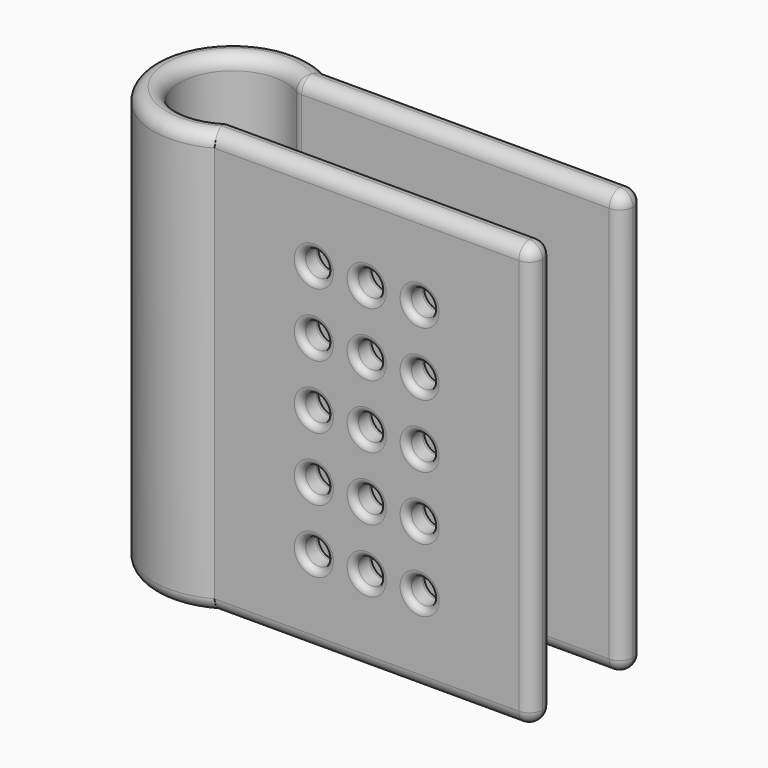
from build123d import *

# Parameters (mm, degrees)
F1_DEPTH = 25.4
F2_R     = 0.79374
F3_R     = 0.79375
F4_DEPTH = 8.9518078406
F5_R     = 0.381


# Not quite as in the source:
# - a fillet or chamfer is up to 0.001 mm smaller than in the source, because OpenCascade refuses the exact size


with BuildPart() as f1:
    # F0 (on Top) → F1 (new body)
    with BuildSketch(Plane.XY):
        with BuildLine():
            ThreePointArc((1.8211051854, -2.6008077406), (-3.175, 0), (1.8211051854, 2.6008077406))
            Line((1.8211051854, 2.6008077406), (2.7316577781, 3.9012116109))
            ThreePointArc((2.7316577781, 3.9012116109), (2.5034693369, 4.0514253701), (2.2670431226, 4.1883077406))
            ThreePointArc((2.2670431226, 4.1883077406), (-4.7625, 0), (2.2670431226, -4.1883077406))
            ThreePointArc((2.2670431226, -4.1883077406), (2.5034693369, -4.0514253701), (2.7316577781, -3.9012116109))
            Line((2.7316577781, -3.9012116109), (1.8211051854, -2.6008077406))
        make_face()
        with BuildLine():
            ThreePointArc((2.2670431226, 4.1883077406), (2.5034693369, 4.0514253701), (2.7316577781, 3.9012116109))
            ThreePointArc((2.7316577781, 3.9012116109), (3.4229686317, 3.3112976303), (3.989637245, 2.6008077406))
            Line((3.989637245, 2.6008077406), (21.3170431226, 2.6008077406))
            Line((21.3170431226, 2.6008077406), (21.3170431226, 4.1883077406))
            Line((21.3170431226, 4.1883077406), (2.2670431226, 4.1883077406))
        make_face()
        with BuildLine():
            Line((3.989637245, -2.6008077406), (1.8211051854, -2.6008077406))
            Line((1.8211051854, -2.6008077406), (2.7316577781, -3.9012116109))
            ThreePointArc((2.7316577781, -3.9012116109), (3.4229686317, -3.3112976303), (3.989637245, -2.6008077406))
        make_face()
        with BuildLine():
            ThreePointArc((3.989637245, -2.6008077406), (3.4229686317, -3.3112976303), (2.7316577781, -3.9012116109))
            ThreePointArc((2.7316577781, -3.9012116109), (2.5034693369, -4.0514253701), (2.2670431226, -4.1883077406))
            Line((2.2670431226, -4.1883077406), (21.3170431226, -4.1883077406))
            Line((21.3170431226, -4.1883077406), (21.3170431226, -2.6008077406))
            Line((21.3170431226, -2.6008077406), (3.989637245, -2.6008077406))
        make_face()
        with BuildLine():
            Line((2.7316577781, 3.9012116109), (1.8211051854, 2.6008077406))
            Line((1.8211051854, 2.6008077406), (3.989637245, 2.6008077406))
            ThreePointArc((3.989637245, 2.6008077406), (3.4229686317, 3.3112976303), (2.7316577781, 3.9012116109))
        make_face()
    extrude(amount=F1_DEPTH)

    # F2 (radius 0.79375 in the source; OpenCascade refuses exactly that, so slightly less here)
    f2_edges = [f1.edges().sort_by_distance(p)[0] for p in [
        (-3.175, 0, 25.4),
        (11.569074, 2.600808, 25.4),
        (21.317043, 3.394558, 25.4),
        (11.792043, 4.188308, 25.4),
        (-4.7625, 0, 25.4),
        (11.792043, -4.188308, 25.4),
        (21.317043, -3.394558, 25.4),
        (11.569074, -2.600808, 25.4),
        (-3.175, 0, 0),
        (11.569074, 2.600808, 0),
        (21.317043, 3.394558, 0),
        (11.792043, 4.188308, 0),
        (-4.7625, 0, 0),
        (11.792043, -4.188308, 0),
        (21.317043, -3.394558, 0),
        (11.569074, -2.600808, 0),
        (21.317043, 2.600808, 12.7),
        (21.317043, 4.188308, 12.7),
        (21.317043, -4.188308, 12.7),
        (21.317043, -2.600808, 12.7),
        (1.821105, -2.600808, 12.7),
        (1.821105, 2.600808, 12.7),
    ]]
    fillet(f2_edges, radius=F2_R)

    # F3 (on face) → F4 (cut, through all)
    with BuildSketch(Plane.XZ.offset(4.1883077406)):
        with Locations((11.3951681226, 12.7)):
            Circle(F3_R)
        with Locations((14.5701681226, 12.7000016774)):
            Circle(F3_R)
        with Locations((8.2201681226, 8.8900020029)):
            Circle(F3_R)
        with Locations((11.3951681226, 8.89)):
            Circle(F3_R)
        with Locations((14.5701681226, 8.8900016774)):
            Circle(F3_R)
        with Locations((11.3951681226, 5.08)):
            Circle(F3_R)
        with Locations((14.5701681226, 5.0800016774)):
            Circle(F3_R)
        with Locations((8.2201681226, 12.7000016774)):
            Circle(F3_R)
        with Locations((11.3951681226, 16.5100008387)):
            Circle(F3_R)
        with Locations((14.5701681226, 16.5100016774)):
            Circle(F3_R)
        with Locations((8.2201681226, 20.3200016774)):
            Circle(F3_R)
        with Locations((11.3951681226, 20.3200016774)):
            Circle(F3_R)
        with Locations((14.5701681226, 20.3200016774)):
            Circle(F3_R)
        with Locations((8.2201681226, 16.5100016774)):
            Circle(F3_R)
        with Locations((8.2201681226, 5.0800023283)):
            Circle(F3_R)
    extrude(amount=-F4_DEPTH, mode=Mode.SUBTRACT)

    # F5
    f5_edges = [f1.edges().sort_by_distance(p)[0] for p in [
        (7.426418, -4.188308, 5.080002),
        (9.013918, -3.394558, 5.080002),
        (7.426418, -2.600808, 5.080002),
        (7.426418, 2.600808, 5.080002),
        (9.013918, 3.394558, 5.080002),
        (7.426418, 4.188308, 5.080002),
        (10.601418, -4.188308, 5.08),
        (12.188918, -3.394558, 5.08),
        (10.601418, -2.600808, 5.08),
        (10.601418, 2.600808, 5.08),
        (12.188918, 3.394558, 5.08),
        (10.601418, 4.188308, 5.08),
        (13.776418, -4.188308, 5.080002),
        (15.363918, -3.394558, 5.080002),
        (13.776418, -2.600808, 5.080002),
        (13.776418, 2.600808, 5.080002),
        (15.363918, 3.394558, 5.080002),
        (13.776418, 4.188308, 5.080002),
        (13.776418, -4.188308, 8.890002),
        (15.363918, -3.394558, 8.890002),
        (13.776418, -2.600808, 8.890002),
        (13.776418, 2.600808, 8.890002),
        (15.363918, 3.394558, 8.890002),
        (13.776418, 4.188308, 8.890002),
        (10.601418, -4.188308, 8.89),
        (12.188918, -3.394558, 8.89),
        (10.601418, -2.600808, 8.89),
        (10.601418, 2.600808, 8.89),
        (12.188918, 3.394558, 8.89),
        (10.601418, 4.188308, 8.89),
        (7.426418, -4.188308, 8.890002),
        (9.013918, -3.394558, 8.890002),
        (7.426418, -2.600808, 8.890002),
        (7.426418, 2.600808, 8.890002),
        (9.013918, 3.394558, 8.890002),
        (7.426418, 4.188308, 8.890002),
        (7.426418, -4.188308, 12.700002),
        (9.013918, -3.394558, 12.700002),
        (7.426418, -2.600808, 12.700002),
        (7.426418, 2.600808, 12.700002),
        (9.013918, 3.394558, 12.700002),
        (7.426418, 4.188308, 12.700002),
        (10.601418, -4.188308, 12.7),
        (12.188918, -3.394558, 12.7),
        (10.601418, -2.600808, 12.7),
        (10.601418, 2.600808, 12.7),
        (12.188918, 3.394558, 12.7),
        (10.601418, 4.188308, 12.7),
        (13.776418, -4.188308, 12.700002),
        (15.363918, -3.394558, 12.700002),
        (13.776418, -2.600808, 12.700002),
        (13.776418, 2.600808, 12.700002),
        (15.363918, 3.394558, 12.700002),
        (13.776418, 4.188308, 12.700002),
        (13.776418, -4.188308, 16.510002),
        (15.363918, -3.394558, 16.510002),
        (13.776418, -2.600808, 16.510002),
        (13.776418, 2.600808, 16.510002),
        (15.363918, 3.394558, 16.510002),
        (13.776418, 4.188308, 16.510002),
        (10.601418, -4.188308, 16.510001),
        (12.188918, -3.394558, 16.510001),
        (10.601418, -2.600808, 16.510001),
        (10.601418, 2.600808, 16.510001),
        (12.188918, 3.394558, 16.510001),
        (10.601418, 4.188308, 16.510001),
        (7.426418, -4.188308, 16.510002),
        (9.013918, -3.394558, 16.510002),
        (7.426418, -2.600808, 16.510002),
        (7.426418, 2.600808, 16.510002),
        (9.013918, 3.394558, 16.510002),
        (7.426418, 4.188308, 16.510002),
        (13.776418, -4.188308, 20.320002),
        (15.363918, -3.394558, 20.320002),
        (13.776418, -2.600808, 20.320002),
        (13.776418, 2.600808, 20.320002),
        (15.363918, 3.394558, 20.320002),
        (13.776418, 4.188308, 20.320002),
        (10.601418, -4.188308, 20.320002),
        (12.188918, -3.394558, 20.320002),
        (10.601418, -2.600808, 20.320002),
        (10.601418, 2.600808, 20.320002),
        (12.188918, 3.394558, 20.320002),
        (10.601418, 4.188308, 20.320002),
        (7.426418, -4.188308, 20.320002),
        (9.013918, -3.394558, 20.320002),
        (7.426418, -2.600808, 20.320002),
        (7.426418, 2.600808, 20.320002),
        (9.013918, 3.394558, 20.320002),
        (7.426418, 4.188308, 20.320002),
    ]]
    fillet(f5_edges, radius=F5_R)


solid = f1.part
